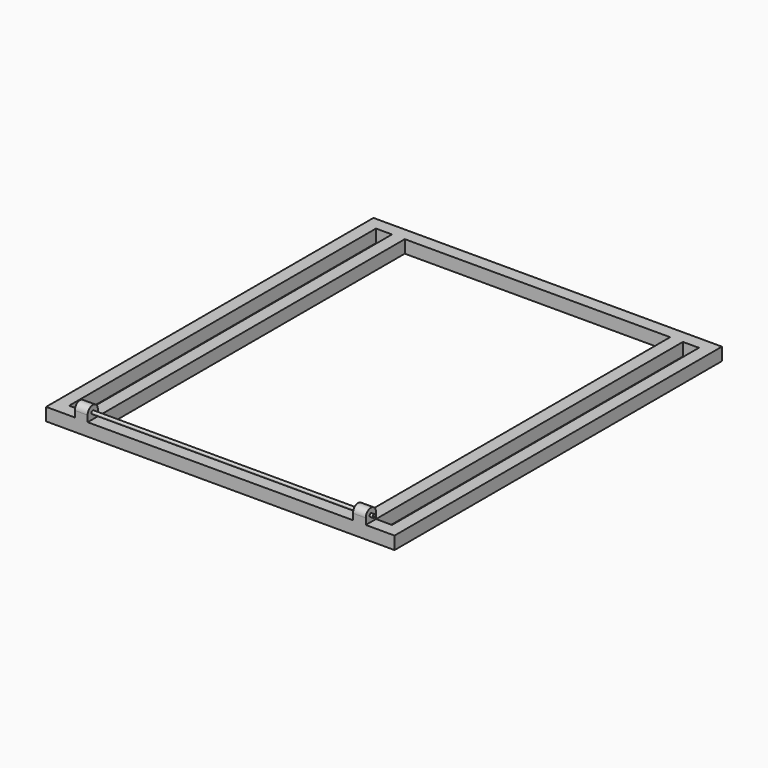
from build123d import *

# Parameters (mm, degrees)
F0_W     = 31.75
F0_H     = 762
F0_W_2   = 527.05
F1_DEPTH = 12.7
F2_R     = 3.175
F3_DEPTH = 25.4
F4_DEPTH = 558.8
F5_DEPTH = 31.75


# Not quite as in the source:
# - a pattern or mirror of a feature is missing from the dataset's text; its kind, count and spacing are read off the source's solid


with BuildPart() as f1:
    # F0 (on Top) → F1 (new body, symmetric)
    with BuildSketch(Plane.XY):
        Polygon((346.075, -12.7), (346.075, 12.7), (-346.075, 12.7), (-346.075, -800.1), (346.075, -800.1), align=None)
        with Locations((-304.8, -393.7)):
            Rectangle(F0_W, F0_H, mode=Mode.SUBTRACT)
        with Locations((0, -393.7)):
            Rectangle(F0_W_2, F0_H, mode=Mode.SUBTRACT)
        with Locations((304.8, -393.7)):
            Rectangle(F0_W, F0_H, mode=Mode.SUBTRACT)
    extrude(amount=F1_DEPTH, both=True)

    # F2 (on face) → F3 (join)
    with BuildSketch(Plane(origin=(263.525, 0, 0), x_dir=(0, -1, 0), z_dir=(-1, 0, 0))):
        with BuildLine():
            Line((800.1, -12.7), (800.1, 12.7))
            Line((800.1, 12.7), (800.1, 25.0216443092))
            ThreePointArc((800.1, 25.0216443092), (787.4, 37.7216443092), (774.7, 25.0216443092))
            Line((774.7, 25.0216443092), (774.7, 12.7))
            Line((774.7, 12.7), (774.7, -12.7))
            Line((774.7, -12.7), (800.1, -12.7))
        make_face()
        with Locations((787.4, 25.0216443092)):
            Circle(F2_R, mode=Mode.SUBTRACT)
    f3 = extrude(amount=-F3_DEPTH)

    # F3_copies: F3 across plane
    add(f3.mirror(Plane(origin=(0, 0, 0), x_dir=(0, 0, -1), z_dir=(-1, 0, 0))))


with BuildPart() as f4:
    # F2 (on face) → F4 (new body)
    with BuildSketch(Plane(origin=(263.525, 0, 0), x_dir=(0, -1, 0), z_dir=(-1, 0, 0))):
        with Locations((787.4, 25.0216443092)):
            Circle(F2_R)
    extrude(amount=F4_DEPTH)

    # F2 (on face) → F5 (join)
    with BuildSketch(Plane(origin=(263.525, 0, 0), x_dir=(0, -1, 0), z_dir=(-1, 0, 0))):
        with Locations((787.4, 25.0216443092)):
            Circle(F2_R)
    extrude(amount=-F5_DEPTH)


solid = Compound([f1.part, f4.part])
